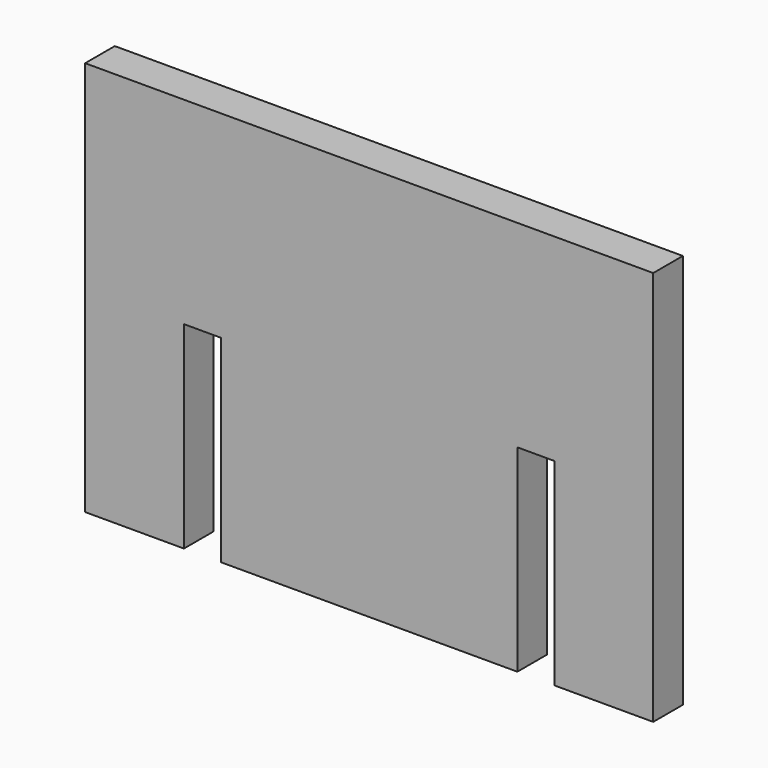
from build123d import *

# Parameters (mm, degrees)
F1_DEPTH = 4.7625


# Not quite as in the source:
# - a length typed as a fraction of an inch, garbled in the dataset ("3 / 203.2 mm" for 3/8 in), is restored


with BuildPart() as f1:
    # F0 (on Front) → F1 (new body)
    with BuildSketch(Plane.XZ):
        Polygon((0, 50.8), (0, 0), (12.7, 0), (12.7, 25.4), (17.4625, 25.4), (17.4625, 0), (55.5625, 0), (55.5625, 25.4), (60.325, 25.4), (60.325, 0), (73.025, 0), (73.025, 50.8), align=None)
    extrude(amount=F1_DEPTH)


solid = f1.part
